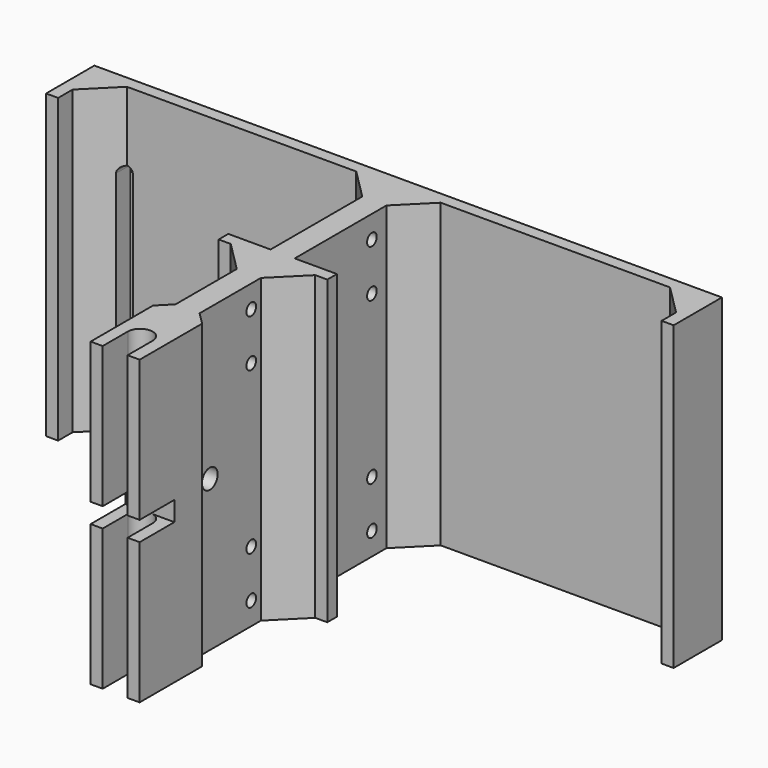
from build123d import *

# Parameters (mm, degrees)
F2_DEPTH     = 50
F3_T1_DEPTH  = 100
F3_T6_DEPTH  = 100
F3_T11_DEPTH = 100
F5_R         = 2
F6_DEPTH     = 8
F8_DEPTH     = 6.001
F9_R         = 3.25
F10_DEPTH    = 25


# Not quite as in the source:
# - a fillet or chamfer that OpenCascade refuses, or shapes differently, is made with other operations: its cross-section is extruded or revolved along the edge and cut away or added


with BuildPart() as f2:
    # F1 (on Top) → F2 (new body, symmetric)
    with BuildSketch(Plane.XY):
        with BuildLine():
            Line((-8.125, 9.6056647934), (-8.125, -10.3943352066))
            Line((-8.125, -10.3943352066), (-4.125, -10.3943352066))
            Line((-4.125, -10.3943352066), (-4.125, 0))
            ThreePointArc((-4.125, 0), (0, 4.125), (4.125, 0))
            Line((4.125, 0), (4.125, -10.3943352066))
            Line((4.125, -10.3943352066), (8.125, -10.3943352066))
            Line((8.125, -10.3943352066), (8.125, 9.6056647934))
            Line((8.125, 9.6056647934), (4, 9.6056647934))
            Line((4, 9.6056647934), (4, 55))
            Line((4, 55), (18, 55))
            Line((18, 55), (18, 59))
            Line((18, 59), (4, 59))
            Line((4, 59), (4, 107))
            Line((4, 107), (100, 107))
            Line((100, 107), (100, 91))
            Line((100, 91), (104, 91))
            Line((104, 91), (104, 111))
            Line((104, 111), (0, 111))
            Line((0, 111), (-104, 111))
            Line((-104, 111), (-104, 91))
            Line((-104, 91), (-100, 91))
            Line((-100, 91), (-100, 107))
            Line((-100, 107), (-4, 107))
            Line((-4, 107), (-4, 59))
            Line((-4, 59), (-18, 59))
            Line((-18, 59), (-18, 55))
            Line((-18, 55), (-4, 55))
            Line((-4, 55), (-4, 9.6056647934))
            Line((-4, 9.6056647934), (-8.125, 9.6056647934))
        make_face()
    extrude(amount=F2_DEPTH, both=True)

    # F3: chamfer of 10 on 8 edges, made by hand

    # F3_s2 → F3_t1 (join)
    with BuildSketch(Plane.XY.offset(-50)):
        Polygon((14, 55), (4, 45), (4, 55), align=None)
        Polygon((-4, 45), (-14, 55), (-4, 55), align=None)
        Polygon((14, 107), (4, 97), (4, 107), align=None)
        Polygon((-4, 97), (-14, 107), (-4, 107), align=None)
        Polygon((100, 97), (90, 107), (100, 107), align=None)
        Polygon((-90, 107), (-100, 97), (-100, 107), align=None)
    extrude(amount=F3_T1_DEPTH)


with BuildPart() as f3_tool4:
    # F3_s5 → F3_t6 (new body)
    with BuildSketch(Plane.XY.offset(-50)):
        Polygon((4, 19.6056647934), (14, 9.6056647934), (4, 9.6056647934), align=None)
    extrude(amount=F3_T6_DEPTH)

    split(bisect_by=Plane.YZ.offset(8.125), keep=Keep.BOTTOM)


with BuildPart() as f2_1:
    add(f2.part)

    # F3_t3: union F3_tool4
    add(f3_tool4.part)


with BuildPart() as f3_tool9:
    # F3_s10 → F3_t11 (new body)
    with BuildSketch(Plane.XY.offset(50)):
        Polygon((-14, 9.6056647934), (-4, 19.6056647934), (-4, 9.6056647934), align=None)
    extrude(amount=-F3_T11_DEPTH)

    split(bisect_by=Plane.YZ.offset(-8.125), keep=Keep.TOP)


with BuildPart() as f2_2:
    add(f2_1.part)

    # F3_t8: union F3_tool9
    add(f3_tool9.part)

    # F5 (on face) → F6 (cut, through all)
    with BuildSketch(Plane(origin=(-4, 0, 0), x_dir=(0, -1, 0), z_dir=(-1, 0, 0))):
        with Locations((-91, -26.75)):
            Circle(F5_R)
        with Locations((-91, -42.5)):
            Circle(F5_R)
        with Locations((-41, -26.75)):
            Circle(F5_R)
        with Locations((-41, -42.5)):
            Circle(F5_R)
        with Locations((-41, 26.75)):
            Circle(F5_R)
        with Locations((-41, 42.5)):
            Circle(F5_R)
        with Locations((-91, 42.5)):
            Circle(F5_R)
        with Locations((-91, 26.75)):
            Circle(F5_R)
    extrude(amount=-F6_DEPTH, mode=Mode.SUBTRACT)

    # F7 (on face) → F8 (cut, through all)
    with BuildSketch(Plane(origin=(0, 111, 0), x_dir=(-1, 0, 0), z_dir=(0, 1, 0))):
        with BuildLine():
            Line((-91.9984134228, 0), (-91.9984134228, -24.9203520777))
            ThreePointArc((-91.9984134228, -24.9203520777), (-89.9790038693, -26.9998897876), (-88.003699271, -24.8784129963))
            Line((-88.003699271, -24.8784129963), (-88.003699271, 0))
            Line((-88.003699271, 0), (-88.003699271, 24.8784129963))
            ThreePointArc((-88.003699271, 24.8784129963), (-89.9790038693, 26.9998897876), (-91.9984134228, 24.9203520777))
            Line((-91.9984134228, 24.9203520777), (-91.9984134228, 0))
        make_face()
        with BuildLine():
            Line((88.003699271, 0), (88.003699271, -24.8784129963))
            ThreePointArc((88.003699271, -24.8784129963), (89.9790038693, -26.9998897876), (91.9984134228, -24.9203520777))
            Line((91.9984134228, -24.9203520777), (91.9984134228, 0))
            Line((91.9984134228, 0), (91.9984134228, 24.9203520777))
            ThreePointArc((91.9984134228, 24.9203520777), (89.9790038693, 26.9998897876), (88.003699271, 24.8784129963))
            Line((88.003699271, 24.8784129963), (88.003699271, 0))
        make_face()
    extrude(amount=-F8_DEPTH, mode=Mode.SUBTRACT)

    # F9 (on face) → F10 (cut)
    with BuildSketch(Plane.YZ.offset(8.125)):
        Polygon((4, 3.25), (-10.3943352066, 3.25), (-10.3943352066, 0), (-10.3943352066, -3.25), (4, -3.25), (4, 0), align=None)
        with Locations((23.8227438553, 0)):
            Circle(F9_R)
    extrude(amount=-F10_DEPTH, mode=Mode.SUBTRACT)


solid = f2_2.part
